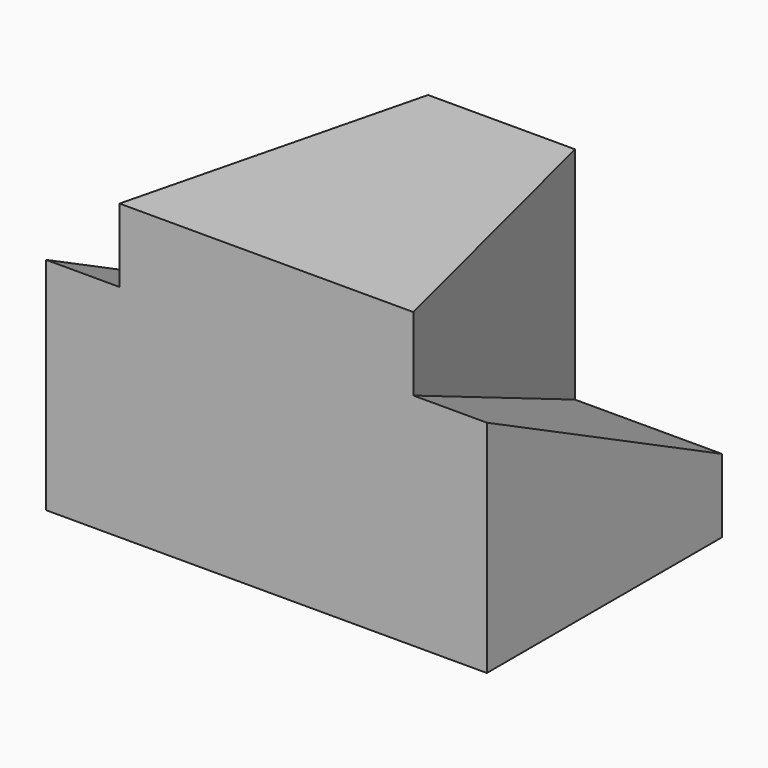
from build123d import *

# Parameters (mm, degrees)
F0_W     = 152.4
F0_H     = 101.6
F1_DEPTH = 76.2
F3_DEPTH = 152.401


with BuildPart() as f1:
    # F0 (on Top) → F1 (new body)
    with BuildSketch(Plane.XY):
        with Locations((76.2, 50.8)):
            Rectangle(F0_W, F0_H)
    extrude(amount=F1_DEPTH)

    # F2 (on face) → F3 (cut, through all)
    with BuildSketch(Plane(origin=(0, 0, 0), x_dir=(0, -1, 0), z_dir=(-1, 0, 0))):
        Polygon((-101.6, 25.4), (0, 76.2), (-101.6, 76.2), align=None)
    extrude(amount=-F3_DEPTH, mode=Mode.SUBTRACT)

    # F6 (on offset) → F7 section 0
    with BuildSketch(Plane.XY.offset(101.6)):
        Polygon((101.6, 101.6), (50.8, 101.6), (25.4, 0), (127, 0), align=None)
    # F4 (on face) → F7 section 1
    with BuildSketch(Plane(origin=(0, 30.48, 60.96), x_dir=(1, 0, 0), z_dir=(0, 0.4472135955, 0.894427191))):
        Polygon((50.8, 79.5145772799), (25.4, -34.0776759771), (127, -34.0776759771), (101.6, 79.5145772799), align=None)
    loft()


solid = f1.part
